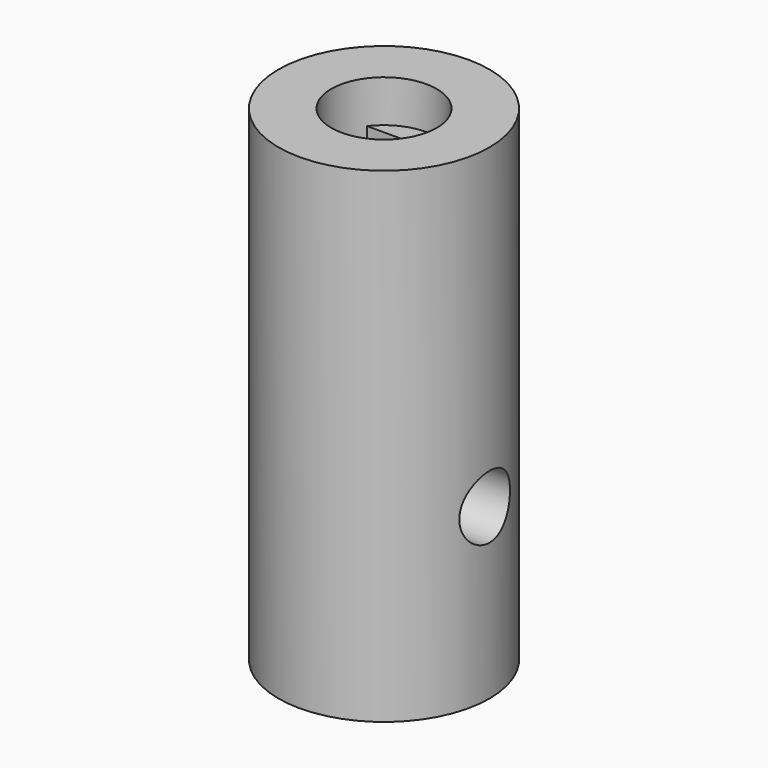
from build123d import *

# Parameters (mm, degrees)
F0_R     = 5
F1_DEPTH = 7
F2_DEPTH = 9
F3_R     = 5
F3_R_2   = 3
F4_DEPTH = 4
F5_DEPTH = 14
F6_R     = 1.5
F7_DEPTH = 12.5


with BuildPart() as f1:
    # F0 (on Top) → F1 (new body)
    with BuildSketch(Plane.XY):
        Circle(F0_R)
        with BuildLine():
            ThreePointArc((-2, 1.5), (0, 2.5), (2, 1.5))
            Line((2, 1.5), (3.6073317751, 1.5))
            Line((3.6073317751, 1.5), (3.6073317751, -1.5))
            Line((3.6073317751, -1.5), (2, -1.5))
            ThreePointArc((2, -1.5), (0, -2.5), (-2, -1.5))
            Line((-2, -1.5), (-3.6073317751, -1.5))
            Line((-3.6073317751, -1.5), (-3.6073317751, 1.5))
            Line((-3.6073317751, 1.5), (-2, 1.5))
        make_face(mode=Mode.SUBTRACT)
        with BuildLine():
            ThreePointArc((2, 1.5), (2.3717082451, 0.790569415), (2.5, 0))
            ThreePointArc((2.5, 0), (2.3717082451, -0.790569415), (2, -1.5))
            Line((2, -1.5), (3.6073317751, -1.5))
            Line((3.6073317751, -1.5), (3.6073317751, 1.5))
            Line((3.6073317751, 1.5), (2, 1.5))
        make_face()
        with BuildLine():
            Line((-2, 1.5), (2, 1.5))
            ThreePointArc((2, 1.5), (0, 2.5), (-2, 1.5))
        make_face()
        with BuildLine():
            ThreePointArc((-2, -1.5), (0, -2.5), (2, -1.5))
            Line((2, -1.5), (-2, -1.5))
        make_face()
        with BuildLine():
            ThreePointArc((-2, -1.5), (-2.5, 0), (-2, 1.5))
            Line((-2, 1.5), (-3.6073317751, 1.5))
            Line((-3.6073317751, 1.5), (-3.6073317751, -1.5))
            Line((-3.6073317751, -1.5), (-2, -1.5))
        make_face()
    extrude(amount=F1_DEPTH)

    # F0 (on Top) → F2 (join)
    with BuildSketch(Plane.XY):
        Circle(F0_R)
        with BuildLine():
            ThreePointArc((-2, 1.5), (0, 2.5), (2, 1.5))
            Line((2, 1.5), (3.6073317751, 1.5))
            Line((3.6073317751, 1.5), (3.6073317751, -1.5))
            Line((3.6073317751, -1.5), (2, -1.5))
            ThreePointArc((2, -1.5), (0, -2.5), (-2, -1.5))
            Line((-2, -1.5), (-3.6073317751, -1.5))
            Line((-3.6073317751, -1.5), (-3.6073317751, 1.5))
            Line((-3.6073317751, 1.5), (-2, 1.5))
        make_face(mode=Mode.SUBTRACT)
        with BuildLine():
            ThreePointArc((-2, -1.5), (-2.5, 0), (-2, 1.5))
            Line((-2, 1.5), (-3.6073317751, 1.5))
            Line((-3.6073317751, 1.5), (-3.6073317751, -1.5))
            Line((-3.6073317751, -1.5), (-2, -1.5))
        make_face()
        with BuildLine():
            ThreePointArc((2, 1.5), (2.3717082451, 0.790569415), (2.5, 0))
            ThreePointArc((2.5, 0), (2.3717082451, -0.790569415), (2, -1.5))
            Line((2, -1.5), (3.6073317751, -1.5))
            Line((3.6073317751, -1.5), (3.6073317751, 1.5))
            Line((3.6073317751, 1.5), (2, 1.5))
        make_face()
    extrude(amount=F2_DEPTH)

    # F3 (on face) → F4 (join)
    with BuildSketch(Plane(origin=(0, 0, 0), x_dir=(1, 0, 0), z_dir=(0, 0, -1))):
        Circle(F3_R)
        Circle(F3_R_2, mode=Mode.SUBTRACT)
        Circle(F3_R_2)
        with BuildLine():
            Line((2, -1.5), (-2, -1.5))
            ThreePointArc((-2, -1.5), (-2.5, 0), (-2, 1.5))
            Line((-2, 1.5), (2, 1.5))
            ThreePointArc((2, 1.5), (2.5, 0), (2, -1.5))
        make_face(mode=Mode.SUBTRACT)
        with BuildLine():
            ThreePointArc((-2, 1.5), (-2.5, 0), (-2, -1.5))
            Line((-2, -1.5), (2, -1.5))
            ThreePointArc((2, -1.5), (2.5, 0), (2, 1.5))
            Line((2, 1.5), (-2, 1.5))
        make_face()
    extrude(amount=F4_DEPTH)

    # F3 (on face) → F5 (join)
    with BuildSketch(Plane(origin=(0, 0, 0), x_dir=(1, 0, 0), z_dir=(0, 0, -1))):
        Circle(F3_R)
        Circle(F3_R_2, mode=Mode.SUBTRACT)
    extrude(amount=F5_DEPTH)

    # F6 (on Right) → F7 (cut, symmetric)
    with BuildSketch(Plane.YZ):
        with Locations((0, -5.9965602363)):
            Circle(F6_R)
    extrude(amount=F7_DEPTH, both=True, mode=Mode.SUBTRACT)


solid = f1.part
